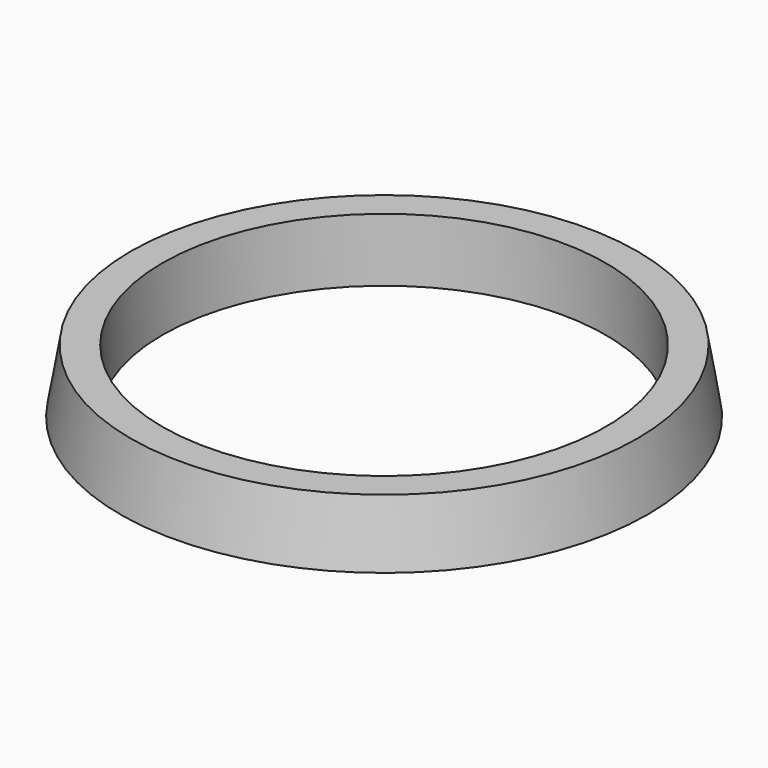
from build123d import *

# Parameters (mm, degrees)
F0_R     = 2.5
F1_DEPTH = 0.6
F2_D     = 4.2
F3_SIZE2 = 0.59999
F3_SIZE  = 0.09999


# Not quite as in the source:
# - a fillet or chamfer is up to 0.001 mm smaller than in the source, because OpenCascade refuses the exact size


with BuildPart() as f1:
    # F0 (on Top) → F1 (new body)
    with BuildSketch(Plane.XY):
        Circle(F0_R)
    extrude(amount=F1_DEPTH)

    # F2 (through all)
    with Locations(Plane(origin=(0, 0, 0), x_dir=(1, 0, 0), z_dir=(0, 0, -1))):
        with Locations((0, 0)):
            Hole(F2_D / 2)

    # F3 (size 0.1 and 0.6 in the source; OpenCascade refuses exactly that, so slightly less here)
    f3_edges = [f1.edges().sort_by_distance(p)[0] for p in [
        (-2.5, 0, 0.6),
    ]]
    f3_side = f1.faces().sort_by_distance((-2.429289, 0, 0.6))[0]
    chamfer(f3_edges, length=F3_SIZE, length2=F3_SIZE2, reference=f3_side)


solid = f1.part
